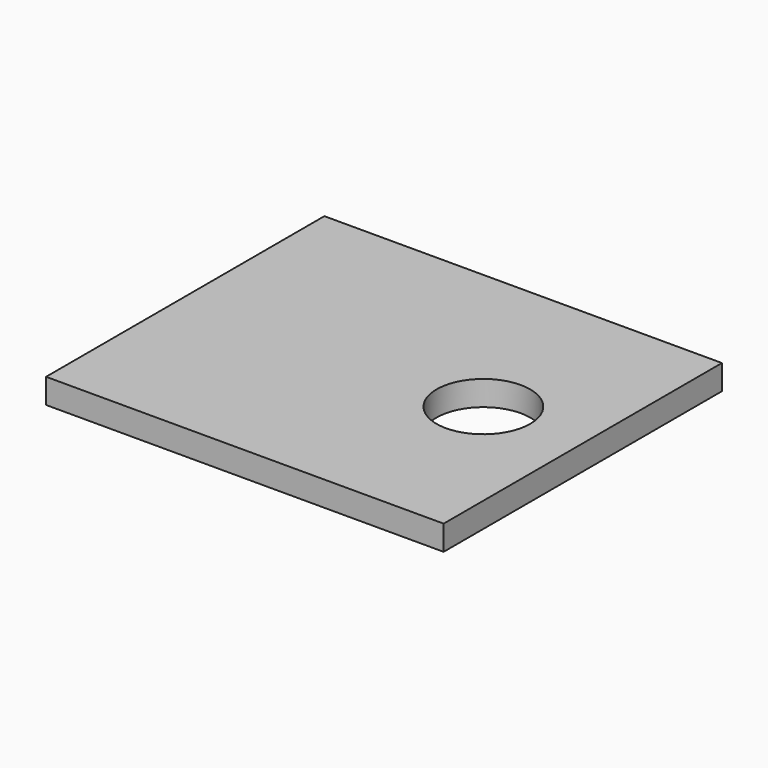
from build123d import *

# Parameters (mm, degrees)
F0_R     = 11.9611676369
F1_DEPTH = 6.35


# Not quite as in the source:
# - a feature names something its author has since deleted; it is built from what else it names


with BuildPart() as f1:
    # F0 (on Top) → F1 (new body)
    with BuildSketch(Plane.XY):
        Polygon((4.9436837435, 38.7340840895), (-45.8563162565, 38.7340840895), (-45.8563162565, -50.1659159105), (55.7436837435, -50.1659159105), (55.7436837435, 38.7340840895), align=None)
        with Locations((30.3436837435, -5.7159159105)):
            Circle(F0_R, mode=Mode.SUBTRACT)
    extrude(amount=F1_DEPTH)


solid = f1.part
